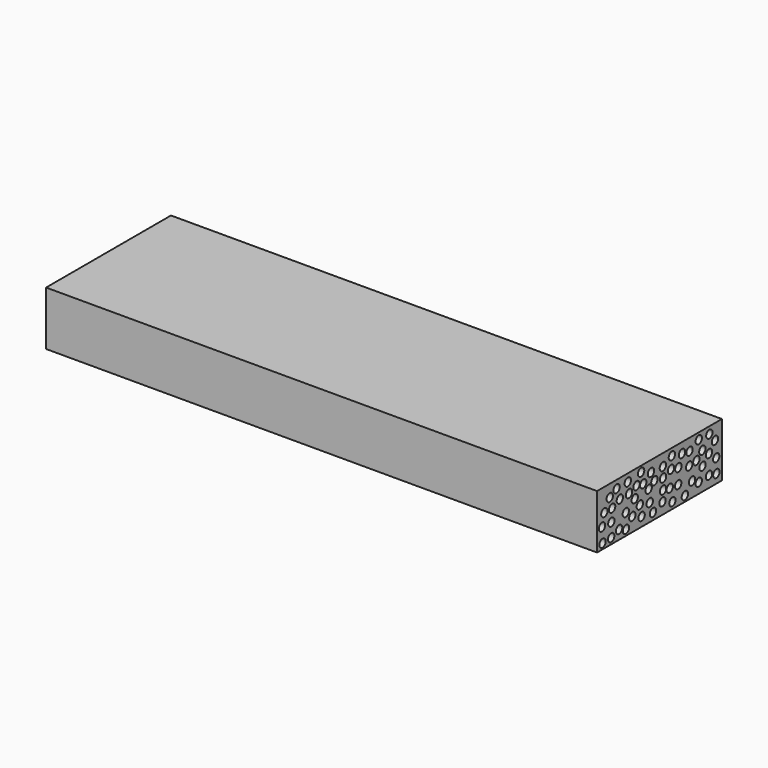
from build123d import *

# Parameters (mm, degrees)
F0_W      = 151.1122360826
F0_H      = 52.3923374712
F0_R      = 3.8560302153
F2_DEPTH  = 508
F3_DEPTH  = 25.4
F2_FACE_W = 151.1122360826
F2_FACE_H = 52.3923374712
F2_FACE_R = 3.8560302153
F4_DEPTH  = 25.4


# Not quite as in the source:
# - the program builds the solid bodies; features that only make, move or delete a surface that nothing else refers to are left out


with BuildPart() as f2:
    # F0 (on Right) → F2 (new body)
    with BuildSketch(Plane.YZ):
        with Locations((-0.8284635842, 35.1436007768)):
            Rectangle(F0_W, F0_H)
        with Locations((-69.7291195393, 14.2931053415)):
            Circle(F0_R, mode=Mode.SUBTRACT)
        with Locations((-59.2672452331, 14.7290164605)):
            Circle(F0_R, mode=Mode.SUBTRACT)
        with Locations((-41.3948856294, 14.511060901)):
            Circle(F0_R, mode=Mode.SUBTRACT)
        with Locations((-70.3829824924, 28.2422658056)):
            Circle(F0_R, mode=Mode.SUBTRACT)
        with Locations((-59.0492933989, 27.8063565493)):
            Circle(F0_R, mode=Mode.SUBTRACT)
        with Locations((-49.6772006154, 17.7803952247)):
            Circle(F0_R, mode=Mode.SUBTRACT)
        with Locations((-41.6128411889, 28.8961324841)):
            Circle(F0_R, mode=Mode.SUBTRACT)
        with Locations((-8.7015386671, 15.6008386984)):
            Circle(F0_R, mode=Mode.SUBTRACT)
        with Locations((-33.7664373219, 22.3574638367)):
            Circle(F0_R, mode=Mode.SUBTRACT)
        with Locations((-22.432744503, 17.7803952247)):
            Circle(F0_R, mode=Mode.SUBTRACT)
        with Locations((-24.6123000979, 28.4602232277)):
            Circle(F0_R, mode=Mode.SUBTRACT)
        with Locations((-12.6247387379, 25.6267972291)):
            Circle(F0_R, mode=Mode.SUBTRACT)
        with Locations((-67.5495639443, 39.3580049276)):
            Circle(F0_R, mode=Mode.SUBTRACT)
        with Locations((-58.1774711609, 39.3580049276)):
            Circle(F0_R, mode=Mode.SUBTRACT)
        with Locations((-48.8053783774, 43.2812049985)):
            Circle(F0_R, mode=Mode.SUBTRACT)
        with Locations((-61.0108934343, 49.6019162238)):
            Circle(F0_R, mode=Mode.SUBTRACT)
        with Locations((-69.9470713735, 55.7046793401)):
            Circle(F0_R, mode=Mode.SUBTRACT)
        with Locations((-52.7285784483, 53.7430755794)):
            Circle(F0_R, mode=Mode.SUBTRACT)
        with Locations((-39.2153263092, 53.9610348642)):
            Circle(F0_R, mode=Mode.SUBTRACT)
        with Locations((-30.7150576264, 36.3066233695)):
            Circle(F0_R, mode=Mode.SUBTRACT)
        with Locations((-37.6896373928, 43.499160558)):
            Circle(F0_R, mode=Mode.SUBTRACT)
        with Locations((-20.4711426049, 44.8068939149)):
            Circle(F0_R, mode=Mode.SUBTRACT)
        with Locations((-13.9324739575, 37.6143604517)):
            Circle(F0_R, mode=Mode.SUBTRACT)
        with Locations((-6.9578932598, 41.9734716415)):
            Circle(F0_R, mode=Mode.SUBTRACT)
        with Locations((-28.5355020314, 46.5505383909)):
            Circle(F0_R, mode=Mode.SUBTRACT)
        with Locations((-23.0866111815, 55.7046793401)):
            Circle(F0_R, mode=Mode.SUBTRACT)
        with Locations((-11.0990498215, 50.6916977465)):
            Circle(F0_R, mode=Mode.SUBTRACT)
        with Locations((14.83767014, 15.1649275795)):
            Circle(F0_R, mode=Mode.SUBTRACT)
        with Locations((29.8766102642, 14.2931053415)):
            Circle(F0_R, mode=Mode.SUBTRACT)
        with Locations((2.8501115739, 19.9599526823)):
            Circle(F0_R, mode=Mode.SUBTRACT)
        with Locations((3.5039787181, 29.767954722)):
            Circle(F0_R, mode=Mode.SUBTRACT)
        with Locations((11.5683367476, 28.0243102461)):
            Circle(F0_R, mode=Mode.SUBTRACT)
        with Locations((21.8122527003, 26.9345343113)):
            Circle(F0_R, mode=Mode.SUBTRACT)
        with Locations((38.5948345065, 23.2292860746)):
            Circle(F0_R, mode=Mode.SUBTRACT)
        with Locations((46.659193933, 18.8701730222)):
            Circle(F0_R, mode=Mode.SUBTRACT)
        with Locations((51.2362644076, 30.6397788227)):
            Circle(F0_R, mode=Mode.SUBTRACT)
        with Locations((59.0826645494, 19.7419971228)):
            Circle(F0_R, mode=Mode.SUBTRACT)
        with Locations((68.0188462138, 17.5624396652)):
            Circle(F0_R, mode=Mode.SUBTRACT)
        with Locations((67.8008943796, 31.0756899416)):
            Circle(F0_R, mode=Mode.SUBTRACT)
        with Locations((3.5039787181, 40.0118716061)):
            Circle(F0_R, mode=Mode.SUBTRACT)
        with Locations((13.0940265954, 43.499160558)):
            Circle(F0_R, mode=Mode.SUBTRACT)
        with Locations((35.1075492799, 37.3964048922)):
            Circle(F0_R, mode=Mode.SUBTRACT)
        with Locations((22.0302101225, 41.3196049631)):
            Circle(F0_R, mode=Mode.SUBTRACT)
        with Locations((3.2860212959, 49.8198717833)):
            Circle(F0_R, mode=Mode.SUBTRACT)
        with Locations((14.1838034615, 54.6148978174)):
            Circle(F0_R, mode=Mode.SUBTRACT)
        with Locations((26.3893213123, 51.5635199845)):
            Circle(F0_R, mode=Mode.SUBTRACT)
        with Locations((35.5434566736, 49.8198717833)):
            Circle(F0_R, mode=Mode.SUBTRACT)
        with Locations((43.8257716596, 38.4861826897)):
            Circle(F0_R, mode=Mode.SUBTRACT)
        with Locations((51.0183051229, 44.3709865212)):
            Circle(F0_R, mode=Mode.SUBTRACT)
        with Locations((59.0826645494, 38.2682271302)):
            Circle(F0_R, mode=Mode.SUBTRACT)
        with Locations((46.659193933, 55.0508089364)):
            Circle(F0_R, mode=Mode.SUBTRACT)
        with Locations((66.2752017379, 46.5505383909)):
            Circle(F0_R, mode=Mode.SUBTRACT)
        with Locations((59.5185756683, 54.6148978174)):
            Circle(F0_R, mode=Mode.SUBTRACT)
        with Locations((-69.9470713735, 55.7046793401)):
            Circle(F0_R)
    extrude(amount=F2_DEPTH)

    # F0 (on Right) → F3 (join)
    with BuildSketch(Plane.YZ):
        with Locations((-61.0108934343, 49.6019162238)):
            Circle(F0_R)
    extrude(amount=F3_DEPTH)

    # F2_face (on face) + F0 (on Right) → F4 (join)
    with BuildSketch(Plane(origin=(508, -0.362148073, 35.2651590305), x_dir=(0, 1, 0), z_dir=(1, 0, 0))):
        with Locations((-0.4663155112, -0.1215582537)):
            Rectangle(F2_FACE_W, F2_FACE_H)
        with Locations((-69.3669714662, -20.972053689)):
            Circle(F2_FACE_R, mode=Mode.SUBTRACT)
        with Locations((-58.90509716, -20.53614257)):
            Circle(F2_FACE_R, mode=Mode.SUBTRACT)
        with Locations((-41.0327375564, -20.7540981295)):
            Circle(F2_FACE_R, mode=Mode.SUBTRACT)
        with Locations((-70.0208344194, -7.0228932249)):
            Circle(F2_FACE_R, mode=Mode.SUBTRACT)
        with Locations((-58.6871453258, -7.4588024812)):
            Circle(F2_FACE_R, mode=Mode.SUBTRACT)
        with Locations((-49.3150525424, -17.4847638058)):
            Circle(F2_FACE_R, mode=Mode.SUBTRACT)
        with Locations((-41.2506931159, -6.3690265464)):
            Circle(F2_FACE_R, mode=Mode.SUBTRACT)
        with Locations((-8.3393905941, -19.664320332)):
            Circle(F2_FACE_R, mode=Mode.SUBTRACT)
        with Locations((-33.4042892489, -12.9076951938)):
            Circle(F2_FACE_R, mode=Mode.SUBTRACT)
        with Locations((-22.07059643, -17.4847638058)):
            Circle(F2_FACE_R, mode=Mode.SUBTRACT)
        with Locations((-24.2501520249, -6.8049358027)):
            Circle(F2_FACE_R, mode=Mode.SUBTRACT)
        with Locations((-12.2625906649, -9.6383618014)):
            Circle(F2_FACE_R, mode=Mode.SUBTRACT)
        with Locations((-67.1874158713, 4.0928458972)):
            Circle(F2_FACE_R, mode=Mode.SUBTRACT)
        with Locations((-57.8153230879, 4.0928458972)):
            Circle(F2_FACE_R, mode=Mode.SUBTRACT)
        with Locations((-48.4432303044, 8.016045968)):
            Circle(F2_FACE_R, mode=Mode.SUBTRACT)
        with Locations((-60.6487453613, 14.3367571933)):
            Circle(F2_FACE_R, mode=Mode.SUBTRACT)
        with Locations((59.8807237414, 19.3497387869)):
            Circle(F2_FACE_R, mode=Mode.SUBTRACT)
        with Locations((-52.3664303753, 18.4779165489)):
            Circle(F2_FACE_R, mode=Mode.SUBTRACT)
        with Locations((-38.8531782362, 18.6958758337)):
            Circle(F2_FACE_R, mode=Mode.SUBTRACT)
        with Locations((-30.3529095533, 1.041464339)):
            Circle(F2_FACE_R, mode=Mode.SUBTRACT)
        with Locations((-37.3274893197, 8.2340015275)):
            Circle(F2_FACE_R, mode=Mode.SUBTRACT)
        with Locations((-20.1089945319, 9.5417348845)):
            Circle(F2_FACE_R, mode=Mode.SUBTRACT)
        with Locations((-13.5703258845, 2.3492014212)):
            Circle(F2_FACE_R, mode=Mode.SUBTRACT)
        with Locations((-6.5957451868, 6.7083126111)):
            Circle(F2_FACE_R, mode=Mode.SUBTRACT)
        with Locations((-28.1733539584, 11.2853793604)):
            Circle(F2_FACE_R, mode=Mode.SUBTRACT)
        with Locations((-22.7244631085, 20.4395203097)):
            Circle(F2_FACE_R, mode=Mode.SUBTRACT)
        with Locations((-10.7369017485, 15.4265387161)):
            Circle(F2_FACE_R, mode=Mode.SUBTRACT)
        with Locations((15.199818213, -20.100231451)):
            Circle(F2_FACE_R, mode=Mode.SUBTRACT)
        with Locations((30.2387583372, -20.972053689)):
            Circle(F2_FACE_R, mode=Mode.SUBTRACT)
        with Locations((3.212259647, -15.3052063482)):
            Circle(F2_FACE_R, mode=Mode.SUBTRACT)
        with Locations((3.8661267911, -5.4972043084)):
            Circle(F2_FACE_R, mode=Mode.SUBTRACT)
        with Locations((11.9304848206, -7.2408487843)):
            Circle(F2_FACE_R, mode=Mode.SUBTRACT)
        with Locations((22.1744007734, -8.3306247192)):
            Circle(F2_FACE_R, mode=Mode.SUBTRACT)
        with Locations((38.9569825795, -12.0358729558)):
            Circle(F2_FACE_R, mode=Mode.SUBTRACT)
        with Locations((47.021342006, -16.3949860083)):
            Circle(F2_FACE_R, mode=Mode.SUBTRACT)
        with Locations((51.5984124807, -4.6253802078)):
            Circle(F2_FACE_R, mode=Mode.SUBTRACT)
        with Locations((59.4448126224, -15.5231619077)):
            Circle(F2_FACE_R, mode=Mode.SUBTRACT)
        with Locations((68.3809942868, -17.7027193653)):
            Circle(F2_FACE_R, mode=Mode.SUBTRACT)
        with Locations((68.1630424526, -4.1894690888)):
            Circle(F2_FACE_R, mode=Mode.SUBTRACT)
        with Locations((3.8661267911, 4.7467125757)):
            Circle(F2_FACE_R, mode=Mode.SUBTRACT)
        with Locations((13.4561746684, 8.2340015275)):
            Circle(F2_FACE_R, mode=Mode.SUBTRACT)
        with Locations((35.469697353, 2.1312458618)):
            Circle(F2_FACE_R, mode=Mode.SUBTRACT)
        with Locations((22.3923581955, 6.0544459326)):
            Circle(F2_FACE_R, mode=Mode.SUBTRACT)
        with Locations((3.648169369, 14.5547127528)):
            Circle(F2_FACE_R, mode=Mode.SUBTRACT)
        with Locations((14.5459515345, 19.3497387869)):
            Circle(F2_FACE_R, mode=Mode.SUBTRACT)
        with Locations((26.7514693853, 16.298360954)):
            Circle(F2_FACE_R, mode=Mode.SUBTRACT)
        with Locations((35.9056047466, 14.5547127528)):
            Circle(F2_FACE_R, mode=Mode.SUBTRACT)
        with Locations((44.1879197326, 3.2210236592)):
            Circle(F2_FACE_R, mode=Mode.SUBTRACT)
        with Locations((51.3804531959, 9.1058274908)):
            Circle(F2_FACE_R, mode=Mode.SUBTRACT)
        with Locations((59.4448126224, 3.0030680997)):
            Circle(F2_FACE_R, mode=Mode.SUBTRACT)
        with Locations((47.021342006, 19.7856499059)):
            Circle(F2_FACE_R, mode=Mode.SUBTRACT)
        with Locations((66.6373498109, 11.2853793604)):
            Circle(F2_FACE_R, mode=Mode.SUBTRACT)
    with BuildSketch(Plane.YZ):
        with Locations((-41.6128411889, 28.8961324841)):
            Circle(F0_R)
        with Locations((-37.6896373928, 43.499160558)):
            Circle(F0_R)
        with Locations((-24.6123000979, 28.4602232277)):
            Circle(F0_R)
        with Locations((38.5948345065, 23.2292860746)):
            Circle(F0_R)
    extrude(amount=F4_DEPTH)


solid = f2.part
